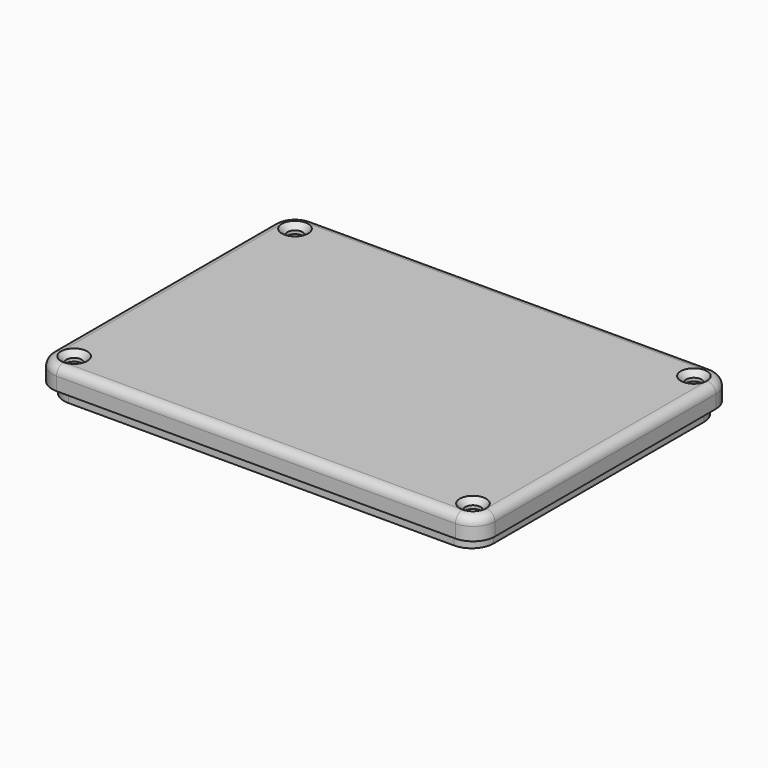
from build123d import *

# Parameters (mm, degrees)
F0_W           = 101
F0_H           = 73
F0_W_2         = 98
F0_H_2         = 70
F0_W_3         = 95
F0_H_3         = 67
F1_DEPTH       = 5
F2_DEPTH       = 3
F3_DEPTH       = 2.5
F4_R           = 2
F5_T1_DEPTH    = 2.5
F5_T3_DEPTH    = 5
F5_T6_ANGLE    = 90
F5_T8_ANGLE    = 90
F5_T10_ANGLE   = 90
F5_T12_ANGLE   = 90
F7_D           = 3.5
F7_DEPTH       = 6
F7_CSINK_D     = 6
F7_CSINK_ANGLE = 90
F7_TIP         = 1.0515060833


# Not quite as in the source:
# - a fillet or chamfer that OpenCascade refuses, or shapes differently, is made with other operations: its cross-section is extruded or revolved along the edge and cut away or added
# - a feature names something its author has since deleted; it is built from what else it names


with BuildPart() as f1:
    # F0 (on Top) → F1 (new body)
    with BuildSketch(Plane.XY):
        Rectangle(F0_W, F0_H)
        Rectangle(F0_W_2, F0_H_2, mode=Mode.SUBTRACT)
        Rectangle(F0_W_2, F0_H_2)
        Rectangle(F0_W_3, F0_H_3, mode=Mode.SUBTRACT)
        Rectangle(F0_W_3, F0_H_3)
    extrude(amount=F1_DEPTH)

    # F0 (on Top) → F2 (cut)
    with BuildSketch(Plane.XY):
        Rectangle(F0_W_3, F0_H_3)
    extrude(amount=F2_DEPTH, mode=Mode.SUBTRACT)

    # F0 (on Top) → F3 (join)
    with BuildSketch(Plane.XY):
        Rectangle(F0_W_2, F0_H_2)
        Rectangle(F0_W_3, F0_H_3, mode=Mode.SUBTRACT)
    extrude(amount=-F3_DEPTH)

    # F4
    f4_edges = [f1.edges().sort_by_distance(p)[0] for p in [
        (-47.5, -33.5, 0.25),
        (-47.5, 33.5, 0.25),
        (47.5, 33.5, 0.25),
        (47.5, -33.5, 0.25),
        (0, -36.5, 5),
        (50.5, 0, 5),
        (-50.5, 0, 5),
        (0, 36.5, 5),
    ]]
    fillet(f4_edges, radius=F4_R)

    # F5: fillet of radius 5 on 8 edges, made by hand

    # F5_s2 → F5_t1 (cut)
    with BuildSketch(Plane.XY.offset(-2.5)):
        with BuildLine():
            ThreePointArc((-44, -35), (-47.5355339059, -33.5355339059), (-49, -30))
            Line((-49, -30), (-49.1, -30))
            Line((-49.1, -30), (-49.1, -35.1))
            Line((-49.1, -35.1), (-44, -35.1))
            Line((-44, -35.1), (-44, -35))
        make_face()
        with BuildLine():
            ThreePointArc((44, -35), (47.5355339059, -33.5355339059), (49, -30))
            Line((49, -30), (49.1, -30))
            Line((49.1, -30), (49.1, -35.1))
            Line((49.1, -35.1), (44, -35.1))
            Line((44, -35.1), (44, -35))
        make_face()
        with BuildLine():
            ThreePointArc((49, 30), (47.5355339059, 33.5355339059), (44, 35))
            Line((44, 35), (44, 35.1))
            Line((44, 35.1), (49.1, 35.1))
            Line((49.1, 35.1), (49.1, 30))
            Line((49.1, 30), (49, 30))
        make_face()
        with BuildLine():
            ThreePointArc((-44, 35), (-47.5355339059, 33.5355339059), (-49, 30))
            Line((-49, 30), (-49.1, 30))
            Line((-49.1, 30), (-49.1, 35.1))
            Line((-49.1, 35.1), (-44, 35.1))
            Line((-44, 35.1), (-44, 35))
        make_face()
    extrude(amount=F5_T1_DEPTH, mode=Mode.SUBTRACT)

    # F5_s4 → F5_t3 (cut)
    with BuildSketch(Plane.XY):
        with BuildLine():
            ThreePointArc((-50.5, -31.5), (-49.0355339059, -35.0355339059), (-45.5, -36.5))
            Line((-45.5, -36.5), (-45.5, -36.6))
            Line((-45.5, -36.6), (-50.6, -36.6))
            Line((-50.6, -36.6), (-50.6, -31.5))
            Line((-50.6, -31.5), (-50.5, -31.5))
        make_face()
        with BuildLine():
            ThreePointArc((50.5, -31.5), (49.0355339059, -35.0355339059), (45.5, -36.5))
            Line((45.5, -36.5), (45.5, -36.6))
            Line((45.5, -36.6), (50.6, -36.6))
            Line((50.6, -36.6), (50.6, -31.5))
            Line((50.6, -31.5), (50.5, -31.5))
        make_face()
        with BuildLine():
            ThreePointArc((45.5, 36.5), (49.0355339059, 35.0355339059), (50.5, 31.5))
            Line((50.5, 31.5), (50.6, 31.5))
            Line((50.6, 31.5), (50.6, 36.6))
            Line((50.6, 36.6), (45.5, 36.6))
            Line((45.5, 36.6), (45.5, 36.5))
        make_face()
        with BuildLine():
            ThreePointArc((-45.5, 36.5), (-49.0355339059, 35.0355339059), (-50.5, 31.5))
            Line((-50.5, 31.5), (-50.6, 31.5))
            Line((-50.6, 31.5), (-50.6, 36.6))
            Line((-50.6, 36.6), (-45.5, 36.6))
            Line((-45.5, 36.6), (-45.5, 36.5))
        make_face()
    extrude(amount=F5_T3_DEPTH, mode=Mode.SUBTRACT)

    # F5_s5 → F5_t6 (revolve, cut)
    with BuildSketch(Plane.YZ.offset(-45.5)):
        with BuildLine():
            ThreePointArc((34.5, 5), (35.9142135624, 4.4142135624), (36.5, 3))
            Line((36.5, 3), (36.5, 5))
            Line((36.5, 5), (34.5, 5))
        make_face()
    revolve(axis=Axis((-45.5, 31.5, 5), (0, 0, 1)), revolution_arc=F5_T6_ANGLE, mode=Mode.SUBTRACT)

    # F5_s7 → F5_t8 (revolve, cut)
    with BuildSketch(Plane.XZ.offset(-31.5)):
        with BuildLine():
            ThreePointArc((48.5, 5), (49.9142135624, 4.4142135624), (50.5, 3))
            Line((50.5, 3), (50.5, 5))
            Line((50.5, 5), (48.5, 5))
        make_face()
    revolve(axis=Axis((45.5, 31.5, 5), (0, 0, 1)), revolution_arc=F5_T8_ANGLE, mode=Mode.SUBTRACT)

    # F5_s9 → F5_t10 (revolve, cut)
    with BuildSketch(Plane.YZ.offset(45.5)):
        with BuildLine():
            ThreePointArc((-34.5, 5), (-35.9142135624, 4.4142135624), (-36.5, 3))
            Line((-36.5, 3), (-36.5, 5))
            Line((-36.5, 5), (-34.5, 5))
        make_face()
    revolve(axis=Axis((45.5, -31.5, 5), (0, 0, 1)), revolution_arc=F5_T10_ANGLE, mode=Mode.SUBTRACT)

    # F5_s11 → F5_t12 (revolve, cut)
    with BuildSketch(Plane.XZ.offset(31.5)):
        with BuildLine():
            ThreePointArc((-48.5, 5), (-49.9142135624, 4.4142135624), (-50.5, 3))
            Line((-50.5, 3), (-50.5, 5))
            Line((-50.5, 5), (-48.5, 5))
        make_face()
    revolve(axis=Axis((-45.5, -31.5, 5), (0, 0, 1)), revolution_arc=F5_T12_ANGLE, mode=Mode.SUBTRACT)

    # F7
    with Locations(Plane.XY.offset(5)):
        with Locations((45.5, -31.5), (-45.5, -31.5), (-45.5, 31.5), (45.5, 31.5)):
            CounterSinkHole(F7_D / 2, F7_CSINK_D / 2, depth=F7_DEPTH, counter_sink_angle=F7_CSINK_ANGLE)
            with Locations((0, 0, -(F7_DEPTH + F7_TIP / 2))):  # 118° drill point
                Cone(0, F7_D / 2, F7_TIP, mode=Mode.SUBTRACT)


solid = f1.part
